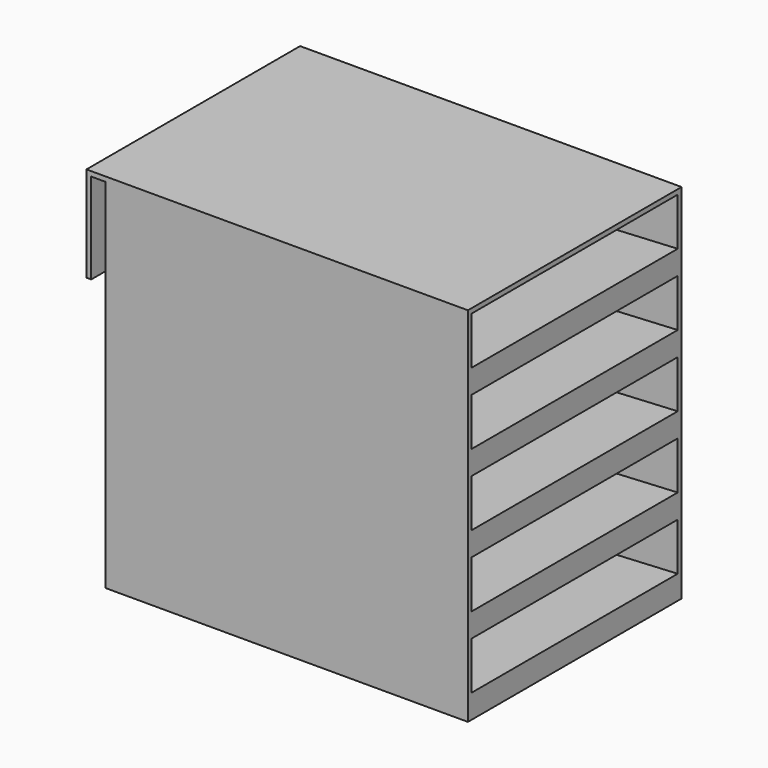
from build123d import *

# Parameters (mm, degrees)
F0_W           = 76
F0_H           = 76
F1_DEPTH       = 28
F2_W           = 54
F2_H           = 10
F5_W           = 56
F5_H           = 76
F6_DEPTH       = 1
F8_DEPTH       = 56
F9_TEXT_SIZE   = 8.9253324808
F9_TEXT_SIZE_2 = 9.2617753479
F9_TEXT_SIZE_3 = 9.3902593815
F9_TEXT_SIZE_4 = 9.6482923254
F9_TEXT_SIZE_5 = 10.8240379228
F10_DEPTH      = 1


# Not quite as in the source:
# - Text() gives the source's letters only with a copy of the font that has no kerning and outlines rounded to 1/6400 em; it was checked with that copy


with BuildPart() as f1:
    # F0 (on Front) → F1 (new body, symmetric)
    with BuildSketch(Plane.XZ):
        Rectangle(F0_W, F0_H)
    extrude(amount=F1_DEPTH, both=True)

    # F4: sweep along a path in F3
    with BuildLine(Plane.XZ.offset(28)) as f4_path:
        Line((38, 37), (-38, 33.0170087745))
    # F2 (on face) → F4 (sweep, cut)
    with BuildSketch(Plane.YZ.offset(38)):
        with Locations((0, 32)):
            Rectangle(F2_W, F2_H)
        with Locations((0, 17)):
            Rectangle(F2_W, F2_H)
        with Locations((0, 2)):
            Rectangle(F2_W, F2_H)
        with Locations((0, -13)):
            Rectangle(F2_W, F2_H)
        with Locations((0, -28)):
            Rectangle(F2_W, F2_H)
    sweep(path=f4_path.line, mode=Mode.SUBTRACT)

    # F5 (on face) → F6 (join)
    with BuildSketch(Plane(origin=(-38, 0, 0), x_dir=(0, -1, 0), z_dir=(-1, 0, 0))):
        Rectangle(F5_W, F5_H)
    extrude(amount=-F6_DEPTH)

    # F7 (on face) → F8 (join)
    with BuildSketch(Plane.XZ.offset(28)):
        Polygon((-38, 37), (-38, 38), (-42, 38), (-42, 18), (-41, 18), (-41, 37), align=None)
    extrude(amount=-F8_DEPTH)

    # F9 (on face) → F10 (join)
    with BuildSketch(Plane(origin=(0, 28, 0), x_dir=(-1, 0, 0), z_dir=(0, 1, 0))):
        with Locations((-30.6668113917, 28.5186786205)):
            Text('M/N', F9_TEXT_SIZE, font='Open Sans', text_align=(TextAlign.LEFT, TextAlign.BOTTOM))
        with Locations((-30.4371416569, 12.921391055)):
            Text('O/P', F9_TEXT_SIZE_2, font='Open Sans', text_align=(TextAlign.LEFT, TextAlign.BOTTOM))
        with Locations((-29.9739278853, -1.6359465662)):
            Text('Q/R', F9_TEXT_SIZE_3, font='Open Sans', text_align=(TextAlign.LEFT, TextAlign.BOTTOM))
        with Locations((-29.9739278853, -16.6555196047)):
            Text('S', F9_TEXT_SIZE_4, font='Open Sans', text_align=(TextAlign.LEFT, TextAlign.BOTTOM))
        with Locations((-29.9739278853, -33.0321379006)):
            Text('T', F9_TEXT_SIZE_5, font='Open Sans', text_align=(TextAlign.LEFT, TextAlign.BOTTOM))
    extrude(amount=F10_DEPTH)


solid = f1.part
